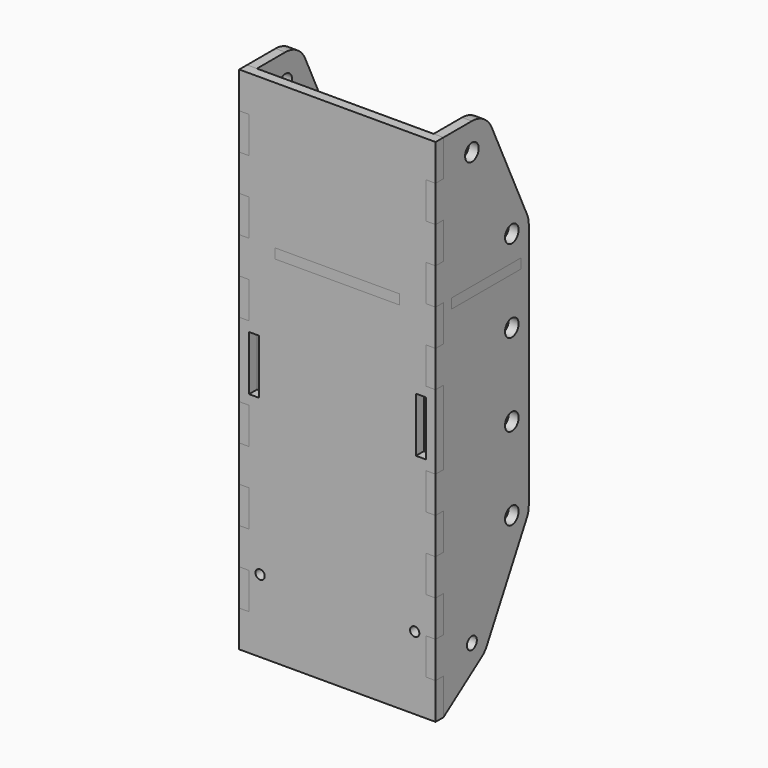
from build123d import *

# Parameters (mm, degrees)
F3_R      = 1.5
F3_W      = 3.175
F3_H      = 17.69
F4_DEPTH  = 3.175
F6_START  = 28.575
F5_R      = 2
F5_R_2    = 2.75
F6_DEPTH  = 3.175
F9_START  = 91.395
F9_DEPTH  = 3.175
F10_START = 91.395
F10_DEPTH = 3.175


# Not quite as in the source:
# - a variable given as a bare number and used for a length is read in inches; the dataset says mm whatever the document's units were


with BuildPart() as f4:
    # F3 (on Front) → F4 (new body)
    with BuildSketch(Plane.XZ):
        Polygon((-31.75, -23.51), (0, -23.51), (31.75, -23.51), (31.75, -11.755), (28.575, -11.755), (28.575, 0), (31.75, 0), (31.75, 11.755), (28.575, 11.755), (28.575, 23.51), (31.75, 23.51), (31.75, 35.265), (28.575, 35.265), (28.575, 47.02), (31.75, 47.02), (31.75, 59.04), (31.75, 71.06), (28.575, 71.06), (28.575, 82.815), (31.75, 82.815), (31.75, 94.57), (28.575, 94.57), (28.575, 106.325), (31.75, 106.325), (31.75, 118.08), (28.575, 118.08), (28.575, 129.835), (31.75, 129.835), (31.75, 141.59), (0, 141.59), (-31.75, 141.59), (-31.75, 129.835), (-28.575, 129.835), (-28.575, 118.08), (-31.75, 118.08), (-31.75, 106.325), (-28.575, 106.325), (-28.575, 94.57), (-31.75, 94.57), (-31.75, 82.815), (-28.575, 82.815), (-28.575, 71.06), (-31.75, 71.06), (-31.75, 59.04), (-31.75, 47.02), (-28.575, 47.02), (-28.575, 35.265), (-31.75, 35.265), (-31.75, 23.51), (-28.575, 23.51), (-28.575, 11.755), (-31.75, 11.755), (-31.75, 0), (-28.575, 0), (-28.575, -11.755), (-31.75, -11.755), align=None)
        with Locations((-25, 0)):
            Circle(F3_R, mode=Mode.SUBTRACT)
        with Locations((-26.9875, 59.04)):
            Rectangle(F3_W, F3_H, mode=Mode.SUBTRACT)
        with Locations((25, 0)):
            Circle(F3_R, mode=Mode.SUBTRACT)
        with Locations((26.9875, 59.04)):
            Rectangle(F3_W, F3_H, mode=Mode.SUBTRACT)
    extrude(amount=F4_DEPTH)


with BuildPart() as f6:
    # F5 (on Right) → F6 (new body)
    with BuildSketch(Plane.YZ.offset(F6_START)):
        with BuildLine():
            Line((0, -11.755), (0, -23.51))
            Line((0, -23.51), (15.4543846839, -12.6031246436))
            ThreePointArc((15.4543846839, -12.6031246436), (16.6264931323, -11.5553520352), (17.5291906941, -10.2681835282))
            Line((17.5291906941, -10.2681835282), (33.6683686113, 19.5055976772))
            ThreePointArc((33.6683686113, 19.5055976772), (34.286747164, 21.0879617874), (34.4971779172, 22.7737812054))
            Line((34.4971779172, 22.7737812054), (34.4971779172, 102.9262187946))
            ThreePointArc((34.4971779172, 102.9262187946), (34.3343497631, 104.4117617775), (33.8535972949, 105.8267628468))
            Line((33.8535972949, 105.8267628468), (19.5557288229, 136.4599645122))
            ThreePointArc((19.5557288229, 136.4599645122), (16.2752494954, 140.1986060209), (11.5, 141.59))
            Line((11.5, 141.59), (0, 141.59))
            Line((0, 141.59), (0, 129.835))
            Line((0, 129.835), (-3.175, 129.835))
            Line((-3.175, 129.835), (-3.175, 118.08))
            Line((-3.175, 118.08), (0, 118.08))
            Line((0, 118.08), (0, 106.325))
            Line((0, 106.325), (-3.175, 106.325))
            Line((-3.175, 106.325), (-3.175, 94.57))
            Line((-3.175, 94.57), (0, 94.57))
            Line((0, 94.57), (0, 82.815))
            Line((0, 82.815), (-3.175, 82.815))
            Line((-3.175, 82.815), (-3.175, 71.06))
            Line((-3.175, 71.06), (0, 71.06))
            Line((0, 71.06), (0, 59.04))
            Line((0, 59.04), (0, 47.02))
            Line((0, 47.02), (-3.175, 47.02))
            Line((-3.175, 47.02), (-3.175, 35.265))
            Line((-3.175, 35.265), (0, 35.265))
            Line((0, 35.265), (0, 23.51))
            Line((0, 23.51), (-3.175, 23.51))
            Line((-3.175, 23.51), (-3.175, 11.755))
            Line((-3.175, 11.755), (0, 11.755))
            Line((0, 11.755), (0, 0))
            Line((0, 0), (-3.175, 0))
            Line((-3.175, 0), (-3.175, -11.755))
            Line((-3.175, -11.755), (0, -11.755))
        make_face()
        with Locations((11.5, -7)):
            Circle(F5_R, mode=Mode.SUBTRACT)
        with Locations((27.6391779172, 22.7737812054)):
            Circle(F5_R_2, mode=Mode.SUBTRACT)
        with Locations((27.6391779172, 49.4912604018)):
            Circle(F5_R_2, mode=Mode.SUBTRACT)
        with Locations((11.5, 132.7)):
            Circle(F5_R_2, mode=Mode.SUBTRACT)
        with Locations((27.6391779172, 76.2087395982)):
            Circle(F5_R_2, mode=Mode.SUBTRACT)
        with Locations((27.6391779172, 102.9262187946)):
            Circle(F5_R_2, mode=Mode.SUBTRACT)
    extrude(amount=F6_DEPTH)


with BuildPart() as f7_1:
    # F7: instance of F6
    add(f6.part.mirror(Plane.YZ))


with BuildPart() as f9_tool:
    # F8 (on Top) → F9 (new body)
    with BuildSketch(Plane.XY.offset(F9_START)):
        Polygon((20.1083333333, 11.5), (0, 11.5), (-20.1083333333, 11.5), (-28.575, 34.4971779172), (-28.575, 31.3221779172), (-31.75, 31.3221779172), (-31.75, 3.175), (-28.575, 3.175), (-28.575, 0), (-20.1083333333, 0), (-20.1083333333, -3.175), (0, -3.175), (20.1083333333, -3.175), (20.1083333333, 0), (28.575, 0), (28.575, 3.175), (31.75, 3.175), (31.75, 31.3221779172), (28.575, 31.3221779172), (28.575, 34.4971779172), align=None)
    extrude(amount=F9_DEPTH)


with BuildPart() as f4_1:
    add(f4.part)

    # F9: cut by f9_tool
    add(f9_tool.part, mode=Mode.SUBTRACT)


with BuildPart() as f6_1:
    add(f6.part)

    # F9: cut by f9_tool
    add(f9_tool.part, mode=Mode.SUBTRACT)


with BuildPart() as f7_1_1:
    add(f7_1.part)

    # F9: cut by f9_tool
    add(f9_tool.part, mode=Mode.SUBTRACT)


with BuildPart() as f10:
    # F8 (on Top) → F10 (new body)
    with BuildSketch(Plane.XY.offset(F10_START)):
        Polygon((20.1083333333, 11.5), (0, 11.5), (-20.1083333333, 11.5), (-28.575, 34.4971779172), (-28.575, 31.3221779172), (-31.75, 31.3221779172), (-31.75, 3.175), (-28.575, 3.175), (-28.575, 0), (-20.1083333333, 0), (-20.1083333333, -3.175), (0, -3.175), (20.1083333333, -3.175), (20.1083333333, 0), (28.575, 0), (28.575, 3.175), (31.75, 3.175), (31.75, 31.3221779172), (28.575, 31.3221779172), (28.575, 34.4971779172), align=None)
    extrude(amount=F10_DEPTH)


solid = Compound([f4_1.part, f6_1.part, f7_1_1.part, f10.part])
